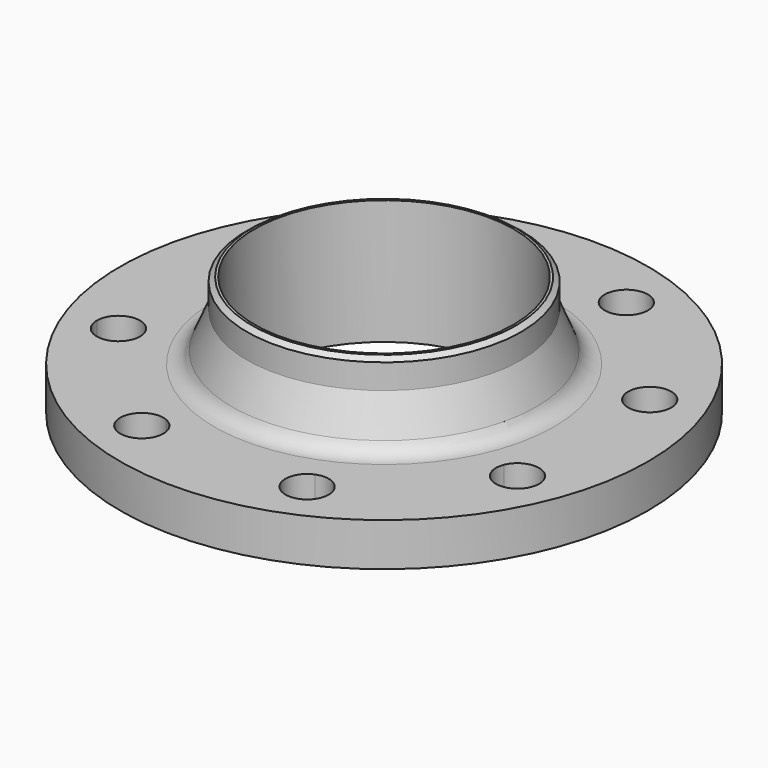
from build123d import *

# Parameters (mm, degrees)
F3_DEPTH        = 20.001
F3_COPIES_COUNT = 8
F6_R            = 8


# Not quite as in the source:
# - a pattern or mirror of a feature is missing from the dataset's text; its kind, count and spacing are read off the source's solid


with BuildPart() as f1:
    # F0 (on Front) → F1 (revolve)
    with BuildSketch(Plane.XZ):
        Polygon((54, 52), (54, 0), (79, 0), (79, 2), (110, 2), (110, 20), (65.5, 20), (57.15, 40), (57.15, 52), align=None)
    revolve(axis=Axis((0, 0, 26), (0, 0, -1)))

    # F2 (on face) → F3 (cut, through all)
    with BuildSketch(Plane.XY.offset(20)):
        with BuildLine():
            ThreePointArc((74.8342421334, 30.9973580216), (84.9049708242, 25.6144413892), (92.149157926, 34.4415089129))
            ThreePointArc((92.149157926, 34.4415089129), (81.3933450279, 43.2685764365), (74.8342421334, 30.9973580216))
        make_face()
    f3 = extrude(amount=-F3_DEPTH, mode=Mode.SUBTRACT)

    # F3_copies: F3 ×8 about axis
    f3_copies_axis = Axis((0, 0, 0), (0, 0, 1))
    for i in range(1, F3_COPIES_COUNT):
        add(f3.rotate(f3_copies_axis, i * 360 / F3_COPIES_COUNT), mode=Mode.SUBTRACT)

    # F4 (on Front) → F5 (revolve, cut)
    with BuildSketch(Plane.XZ):
        Polygon((57.15, 52), (55, 52), (55, 51.999), (57.15, 50.3492469758), align=None)
    revolve(axis=Axis((0, 0, 26), (0, 0, -1)), mode=Mode.SUBTRACT)

    # F6
    f6_edges = [f1.edges().sort_by_distance(p)[0] for p in [
        (-65.5, 0, 20),
    ]]
    fillet(f6_edges, radius=F6_R)


solid = f1.part
